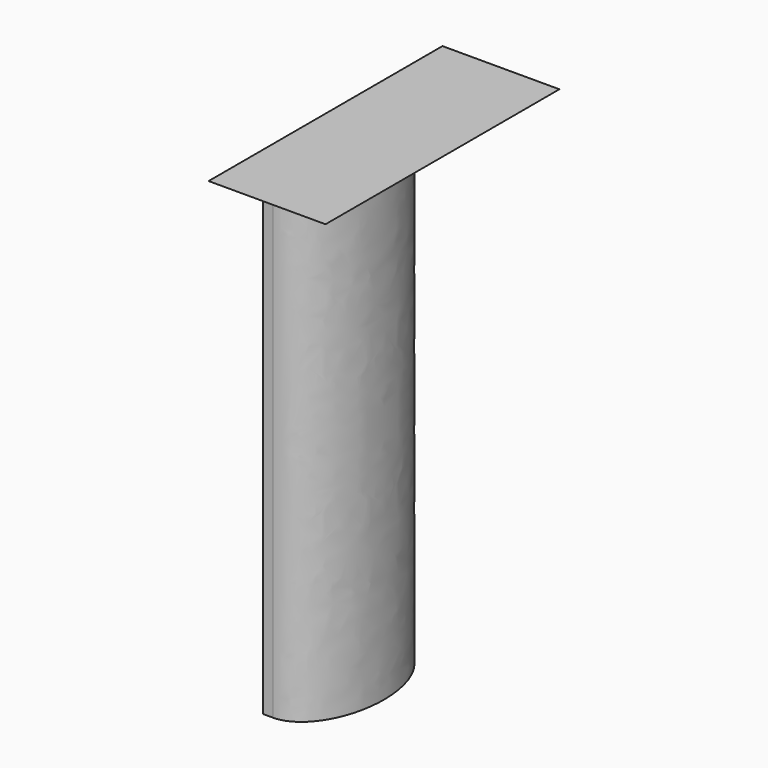
from build123d import *

# Parameters (mm, degrees)
F1_DEPTH = 250
F3_DEPTH = 5
F4_SIZE2 = 4.99999
F4_SIZE  = 9.99999
F6_DEPTH = 240


# Not quite as in the source:
# - a fillet or chamfer is up to 0.001 mm smaller than in the source, because OpenCascade refuses the exact size
# - a feature names something its author has since deleted; it is built from what else it names


with BuildPart() as f1:
    # F0 (on Top) → F1 (new body)
    with BuildSketch(Plane.XY):
        with BuildLine():
            Line((1.0000000522, -46.1442264915), (6.0000000522, -46.1442264915))
            add(Edge.make_bspline(
                [(6, -46.1442264915), (31, -46.1442264915), (31, -6.1442264915), (31, 33.8557735085), (6, 33.8557735085)],
                knots=[0, 0, 0, 1.5707963268, 1.5707963268, 3.1415926536, 3.1415926536, 3.1415926536], degree=2, weights=[1, 0.7071067812, 1, 0.7071067812, 1]))
            Line((6.0000000522, 33.8557735085), (1.0000000522, 33.8557735085))
            Line((1.0000000522, 33.8557735085), (1.0000000522, -46.1442264915))
        make_face()
    extrude(amount=F1_DEPTH)

    # F2 (on face) → F3 (join)
    with BuildSketch(Plane.XY.offset(250)):
        with BuildLine():
            Line((61.0000000522, -81.1442264915), (61.0000000522, 68.8557735085))
            Line((61.0000000522, 68.8557735085), (1.0000000522, 68.8557735085))
            Line((1.0000000522, 68.8557735085), (1.0000000522, 33.8557735085))
            Line((1.0000000522, 33.8557735085), (6.0000000522, 33.8557735085))
            add(Edge.make_bspline(
                [(6, -46.1442264915), (31, -46.1442264915), (31, -6.1442264915), (31, 33.8557735085), (6, 33.8557735085)],
                knots=[0, 0, 0, 1.5707963268, 1.5707963268, 3.1415926536, 3.1415926536, 3.1415926536], degree=2, weights=[1, 0.7071067812, 1, 0.7071067812, 1]))
            Line((6.0000000522, -46.1442264915), (1.0000000522, -46.1442264915))
            Line((1.0000000522, -46.1442264915), (1.0000000522, -81.1442264915))
            Line((1.0000000522, -81.1442264915), (61.0000000522, -81.1442264915))
        make_face()
        with BuildLine():
            Line((6.0000000522, 33.8557735085), (1.0000000522, 33.8557735085))
            Line((1.0000000522, 33.8557735085), (1.0000000522, -46.1442264915))
            Line((1.0000000522, -46.1442264915), (6.0000000522, -46.1442264915))
            add(Edge.make_bspline(
                [(6, -46.1442264915), (31, -46.1442264915), (31, -6.1442264915), (31, 33.8557735085), (6, 33.8557735085)],
                knots=[0, 0, 0, 1.5707963268, 1.5707963268, 3.1415926536, 3.1415926536, 3.1415926536], degree=2, weights=[1, 0.7071067812, 1, 0.7071067812, 1]))
        make_face()
    extrude(amount=F3_DEPTH)

    # F4 (size 10 and 5 in the source; OpenCascade refuses exactly that, so slightly less here)
    f4_edges = [f1.edges().sort_by_distance(p)[0] for p in [
        (31, 68.855774, 250),
        (61, -6.144226, 250),
        (31, -81.144226, 250),
    ]]
    f4_side = f1.faces().sort_by_distance((35.795895, -6.144226, 250))[0]
    chamfer(f4_edges, length=F4_SIZE, length2=F4_SIZE2, reference=f4_side)

    # F5 (on face) → F6 (cut)
    with BuildSketch(Plane(origin=(0, 0, 0), x_dir=(1, 0, 0), z_dir=(0, 0, -1))):
        with BuildLine():
            Line((3.5000000522, -23.8557735085), (6.0000000522, -23.8557735085))
            add(Edge.make_bspline(
                [(6, -23.8557735085), (24.75, -23.8557735085), (24.75, 6.1442264915), (24.75, 36.1442264915), (6, 36.1442264915)],
                knots=[0, 0, 0, 1.5707963268, 1.5707963268, 3.1415926536, 3.1415926536, 3.1415926536], degree=2, weights=[1, 0.7071067812, 1, 0.7071067812, 1]))
            Line((6.0000000522, 36.1442264915), (3.5000000522, 36.1442264915))
            Line((3.5000000522, 36.1442264915), (2.0000000522, 36.1442264915))
            Line((2.0000000522, 36.1442264915), (1.0000000522, 36.1442264915))
            Line((1.0000000522, 36.1442264915), (1.0000000522, 6.1442264915))
            Line((1.0000000522, 6.1442264915), (1.0000000522, -23.8557735085))
            Line((1.0000000522, -23.8557735085), (2.0000000522, -23.8557735085))
            Line((2.0000000522, -23.8557735085), (3.5000000522, -23.8557735085))
        make_face()
        Polygon((6.0000000522, -28.8557735085), (6.0000000522, -23.8557735085), (3.5000000522, -23.8557735085), (2.0000000522, -23.8557735085), (2.0000000522, -28.8557735085), align=None)
        Polygon((3.5000000522, 36.1442264915), (6.0000000522, 36.1442264915), (6.0000000522, 41.1442264915), (2.0000000522, 41.1442264915), (2.0000000522, 36.1442264915), align=None)
    extrude(amount=-F6_DEPTH, mode=Mode.SUBTRACT)


solid = f1.part
